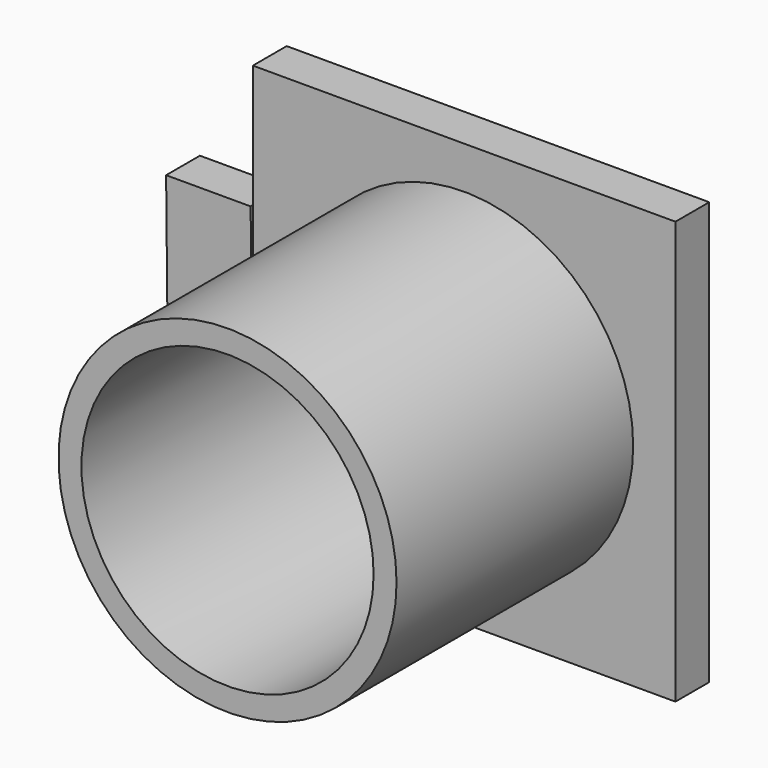
from build123d import *

# Parameters (mm, degrees)
F0_R     = 25.4
F0_R_2   = 21.9544919018
F1_DEPTH = 50.8
F2_DEPTH = 114
F3_W     = 63.5
F3_H     = 63.5
F4_DEPTH = 6.35
F6_DEPTH = 6.35


# Not quite as in the source:
# - an extrude ends at something that could not be found from the text; its depth is read off the source's solid


with BuildPart() as f1:
    # F0 (on Front) → F1 (new body)
    with BuildSketch(Plane.XZ):
        Circle(F0_R)
        Circle(F0_R_2, mode=Mode.SUBTRACT)
    extrude(amount=F1_DEPTH)

    # F0 (on Front) → F2 (cut, through all)
    with BuildSketch(Plane.XZ):
        Circle(F0_R_2)
    extrude(amount=-F2_DEPTH, mode=Mode.SUBTRACT)

    # F3 (on Front) → F4 (join)
    with BuildSketch(Plane.XZ):
        Rectangle(F3_W, F3_H)
    extrude(amount=F4_DEPTH)


with BuildPart() as f6:
    # F5 (on Front) → F6 (new body)
    with BuildSketch(Plane.XZ):
        Polygon((-31.7943245173, -15.7453678548), (-32.0894233882, 13.013583608), (-44.7894233882, 13.013583608), (-44.4943245173, -15.7453678548), align=None)
    extrude(amount=F6_DEPTH)


solid = Compound([f1.part, f6.part])
